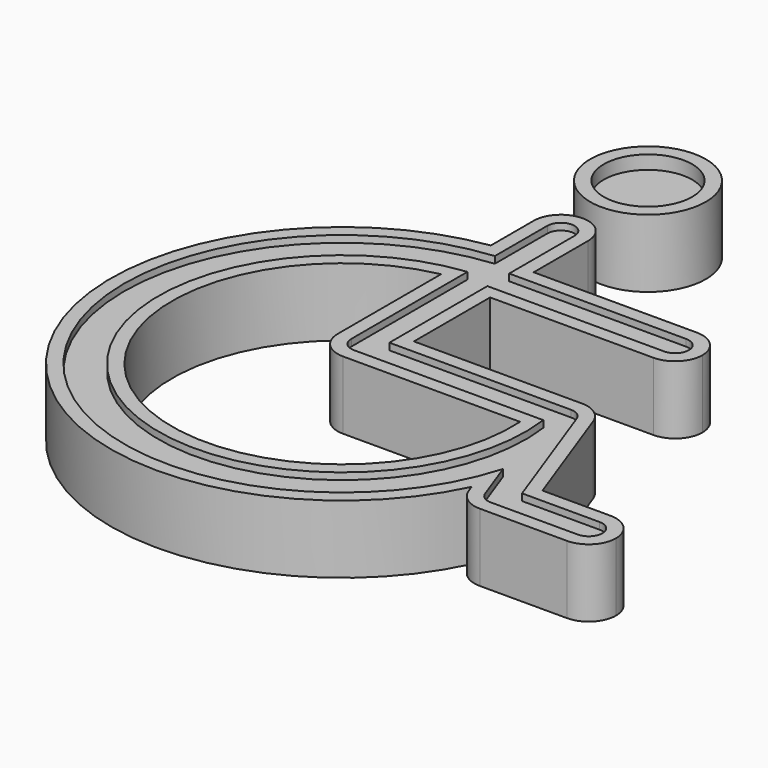
from build123d import *

# Parameters (mm, degrees)
F1_DEPTH = 5
F0_R     = 4.25
F2_R     = 1.99999
F3_R     = 3.25
F4_DEPTH = 0.5
F5_R     = 1
F6_R     = 3.25
F7_DEPTH = 1


# Not quite as in the source:
# - a fillet or chamfer is up to 0.001 mm smaller than in the source, because OpenCascade refuses the exact size


with BuildPart() as f1:
    # F0 (on Top) → F1 (new body)
    with BuildSketch(Plane.XY):
        with BuildLine():
            Line((35.8289553412, 21.6151545151), (22.0794297924, 21.6151545151))
            Line((22.0794297924, 21.6151545151), (22.0794297924, 28.6151545151))
            Line((22.0794297924, 28.6151545151), (36.0794297924, 28.6151545151))
            Line((36.0794297924, 28.6151545151), (36.0794297924, 32.6151545151))
            Line((36.0794297924, 32.6151545151), (22.0794297924, 32.6151545151))
            Line((22.0794297924, 32.6151545151), (22.0794297924, 39.6151545151))
            Line((22.0794297924, 39.6151545151), (18.0794297924, 39.6151545151))
            Line((18.0794297924, 39.6151545151), (18.0794297924, 33.6841086822))
            ThreePointArc((18.0794297924, 33.6841086822), (6.9453736492, 6.7475398575), (35.9550171357, 9.5735849806))
            Line((35.9550171357, 9.5735849806), (36.6193366933, 7.7483819969))
            Line((36.6193366933, 7.7483819969), (46.4201668461, 7.7483819969))
            Line((46.4201668461, 7.7483819969), (46.4201668461, 11.7483819969))
            Line((46.4201668461, 11.7483819969), (39.4201668461, 11.7483819969))
            Line((39.4201668461, 11.7483819969), (35.8289553412, 21.6151545151))
        make_face()
        with BuildLine():
            ThreePointArc((33.0794297924, 17.6151545151), (12.9961320833, 6.9521575032), (18.0794297924, 29.1151545151))
            Line((18.0794297924, 29.1151545151), (18.0794297924, 17.6151545151))
            Line((18.0794297924, 17.6151545151), (33.0794297924, 17.6151545151))
        make_face(mode=Mode.SUBTRACT)
    extrude(amount=F1_DEPTH)

    # F2 (radius 2 in the source; OpenCascade refuses exactly that, so slightly less here)
    f2_edges = [f1.edges().sort_by_distance(p)[0] for p in [
        (18.07943, 39.615155, 2.5),
        (22.07943, 39.615155, 2.5),
        (35.828955, 21.615155, 2.5),
        (36.07943, 28.615155, 2.5),
        (36.07943, 32.615155, 2.5),
        (46.420167, 11.748382, 2.5),
        (46.420167, 7.748382, 2.5),
        (18.07943, 17.615155, 2.5),
        (36.619337, 7.748382, 2.5),
    ]]
    fillet(f2_edges, radius=F2_R)


with BuildPart() as f1b:
    # F0 (on Top) → F1, piece 2 (new body)
    with BuildSketch(Plane.XY):
        with Locations((20.0794297924, 45.6151545151)):
            Circle(F0_R)
    extrude(amount=F1_DEPTH)


with BuildPart() as f4_tool:
    # F3 (on face) → F4 (new body)
    with BuildSketch(Plane.XY.offset(5)):
        with BuildLine():
            Line((19.0794297924, 37.6151545151), (19.0794297924, 32.799673159))
            ThreePointArc((19.0794297924, 32.799673159), (8.2893286135, 6.654126324), (35.975610287, 12.4408101625))
            Line((35.975610287, 12.4408101625), (37.0800591489, 9.4063618536))
            ThreePointArc((37.0800591489, 9.4063618536), (37.4461753333, 8.9292299526), (38.0197517697, 8.7483819969))
            Line((38.0197517697, 8.7483819969), (44.4201668461, 8.7483819969))
            ThreePointArc((44.4201668461, 8.7483819969), (45.4201668461, 9.7483819969), (44.4201668461, 10.7483819969))
            Line((44.4201668461, 10.7483819969), (38.7199593079, 10.7483819969))
            Line((38.7199593079, 10.7483819969), (35.3682328855, 19.9571746585))
            ThreePointArc((35.3682328855, 19.9571746585), (35.0021167011, 20.4343065594), (34.4285402648, 20.6151545151))
            Line((34.4285402648, 20.6151545151), (21.0794297924, 20.6151545151))
            Line((21.0794297924, 20.6151545151), (21.0794297924, 29.6151545151))
            Line((21.0794297924, 29.6151545151), (34.0794297924, 29.6151545151))
            ThreePointArc((34.0794297924, 29.6151545151), (35.0794297924, 30.6151545151), (34.0794297924, 31.6151545151))
            Line((34.0794297924, 31.6151545151), (21.0794297924, 31.6151545151))
            Line((21.0794297924, 31.6151545151), (21.0794297924, 37.6151545151))
            ThreePointArc((21.0794297924, 37.6151545151), (20.0794297924, 38.6151545151), (19.0794297924, 37.6151545151))
        make_face()
        with BuildLine():
            ThreePointArc((33.9885439185, 18.6151545151), (12.2800387641, 6.2419574428), (19.0794297924, 30.2861559837))
            Line((19.0794297924, 30.2861559837), (19.0794297924, 18.6151545151))
            Line((19.0794297924, 18.6151545151), (33.9885439185, 18.6151545151))
        make_face(mode=Mode.SUBTRACT)
        with Locations((20.0794297924, 45.6151545151)):
            Circle(F3_R)
    extrude(amount=-F4_DEPTH)


with BuildPart() as f1_1:
    add(f1.part)

    # F4: cut by f4_tool
    add(f4_tool.part, mode=Mode.SUBTRACT)

    # F5
    f5_edges = [f1_1.edges().sort_by_distance(p)[0] for p in [
        (19.07943, 18.615155, 4.75),
    ]]
    fillet(f5_edges, radius=F5_R)


with BuildPart() as f1b_1:
    add(f1b.part)

    # F4: cut by f4_tool
    add(f4_tool.part, mode=Mode.SUBTRACT)

    # F6 (on face) → F7 (cut)
    with BuildSketch(Plane.XY.offset(5)):
        with Locations((20.0794297924, 45.6151545151)):
            Circle(F6_R)
    extrude(amount=-F7_DEPTH, mode=Mode.SUBTRACT)


solid = Compound([f1_1.part, f1b_1.part])
